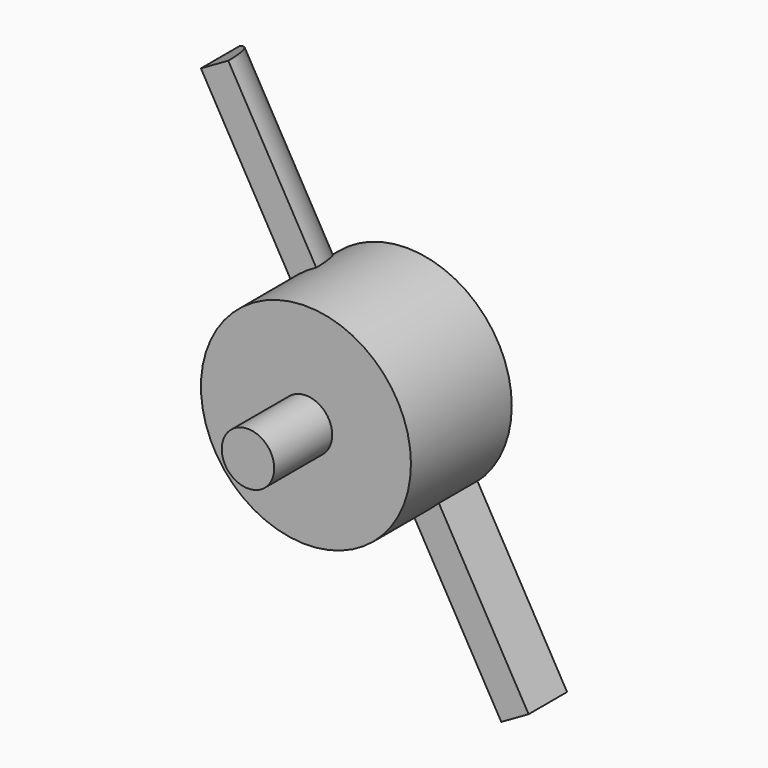
from build123d import *

# Parameters (mm, degrees)
F0_R         = 10
F1_DEPTH     = 12
F3_DEPTH     = 5
F4_T4_DEPTH  = 41.8533803035
F4_S5_R      = 10
F4_T6_DEPTH  = 25
F4_T10_DEPTH = 41.8533803035
F4_S11_R     = 10
F4_T12_DEPTH = 25
F5_R         = 2.5
F6_DEPTH     = 6.9


# Not quite as in the source:
# - a fillet or chamfer that OpenCascade refuses, or shapes differently, is made with other operations: its cross-section is extruded or revolved along the edge and cut away or added


with BuildPart() as f1:
    # F0 (on Front) → F1 (new body)
    with BuildSketch(Plane.XZ):
        Circle(F0_R)
    extrude(amount=F1_DEPTH)

    # F2 (on face) → F3 (join)
    with BuildSketch(Plane(origin=(0, 0, 0), x_dir=(-1, 0, 0), z_dir=(0, 1, 0))):
        Polygon((2.4069448783, 5), (-2.4069448783, 5), (-3, 0), (3, 0), (15.6031129395, 22), (13, 23.4912421078), align=None)
        Polygon((3, 0), (-3, 0), (-15.6031129395, -22), (-13, -23.4912421078), (-2.4069448783, -5), (2.4069448783, -5), align=None)
    extrude(amount=-F3_DEPTH)

    # F4: fillet of radius 5 on 2 edges, made by hand


with BuildPart() as f4_tool2:
    # F4_s3 → F4_t4 (new body)
    with BuildSketch(Plane(origin=(-19.5578893967, 0, 34.1402611236), x_dir=(0, 1, 0), z_dir=(0.4970807026, 0, -0.8677043132))):
        with BuildLine():
            ThreePointArc((0, -4.6031129395), (-1.4644660941, -1.0675790336), (-5, 0.3968870605))
            Line((-5, 0.3968870605), (0, 0.3968870605))
            Line((0, 0.3968870605), (0, -4.6031129395))
        make_face()
    extrude(amount=F4_T4_DEPTH)

    # F4_s5 → F4_t6 (cut, symmetric)
    with BuildSketch(Plane.XZ.offset(2.5)):
        Circle(F4_S5_R)
    extrude(amount=F4_T6_DEPTH, both=True, mode=Mode.SUBTRACT)


with BuildPart() as f1_1:
    add(f1.part)

    # F4_t1: cut F4_tool2
    add(f4_tool2.part, mode=Mode.SUBTRACT)


with BuildPart() as f4_tool8:
    # F4_s9 → F4_t10 (new body)
    with BuildSketch(Plane(origin=(19.5578893967, 0, -34.1402611236), x_dir=(0, 1, 0), z_dir=(-0.4970807026, 0, 0.8677043132))):
        with BuildLine():
            ThreePointArc((0, -4.6031129395), (-1.4644660941, -1.0675790336), (-5, 0.3968870605))
            Line((-5, 0.3968870605), (0, 0.3968870605))
            Line((0, 0.3968870605), (0, -4.6031129395))
        make_face()
    extrude(amount=F4_T10_DEPTH)

    # F4_s11 → F4_t12 (cut, symmetric)
    with BuildSketch(Plane.XZ.offset(2.5)):
        Circle(F4_S11_R)
    extrude(amount=F4_T12_DEPTH, both=True, mode=Mode.SUBTRACT)


with BuildPart() as f1_2:
    add(f1_1.part)

    # F4_t7: cut F4_tool8
    add(f4_tool8.part, mode=Mode.SUBTRACT)

    # F5 (on face) → F6 (join)
    with BuildSketch(Plane.XZ.offset(12)):
        Circle(F5_R)
    extrude(amount=F6_DEPTH)


solid = f1_2.part
